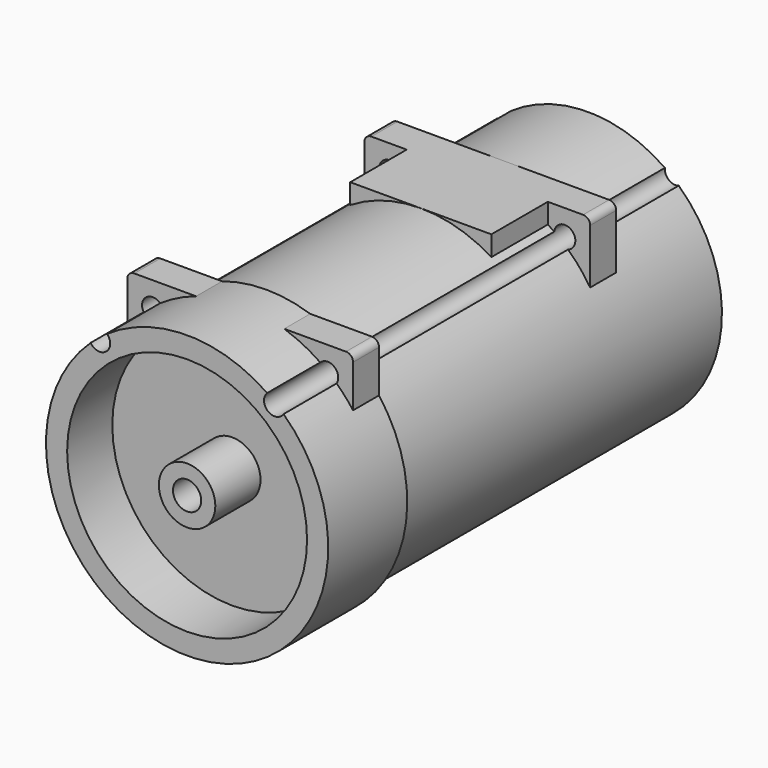
from build123d import *

# Parameters (mm, degrees)
F0_R      = 95
F1_DEPTH  = 355
F3_DEPTH  = 70
F4_R      = 85
F4_R_2    = 20
F5_DEPTH  = 40
F6_R      = 10
F7_DEPTH  = 25
F10_DEPTH = 98
F11_R     = 100
F11_R_2   = 95
F12_DEPTH = 70
F8_R      = 7.5
F13_DEPTH = 500
F14_R     = 5
F16_DEPTH = 47
F18_DEPTH = 75
F19_W     = 100
F19_H     = 50
F20_DEPTH = 22


# Not quite as in the source:
# - a feature names something its author has since deleted; it is built from what else it names


with BuildPart() as f1:
    # F0 (on Front) → F1 (new body)
    with BuildSketch(Plane.XZ):
        Circle(F0_R)
    extrude(amount=F1_DEPTH)

    # F2 (on face) → F3 (join)
    with BuildSketch(Plane.XZ.offset(355)):
        with BuildLine():
            Line((80, 51.2347538298), (80, 95))
            Line((80, 95), (46.4354390525, 95))
            Line((46.4354390525, 95), (0, 95))
            ThreePointArc((0, 95), (45.594398703, 83.3435708793), (80, 51.2347538298))
        make_face()
        with BuildLine():
            ThreePointArc((95, 0), (91.1729126441, 26.6926956301), (80, 51.2347538298))
            Line((80, 51.2347538298), (80, 50))
            Line((80, 50), (-80, 50))
            Line((-80, 50), (-80, 51.2347538298))
            ThreePointArc((-80, 51.2347538298), (-26.6926956301, -91.1729126441), (95, 0))
        make_face()
        with BuildLine():
            Line((80, 50), (80, 51.2347538298))
            ThreePointArc((80, 51.2347538298), (45.594398703, 83.3435708793), (0, 95))
            ThreePointArc((0, 95), (-45.594398703, 83.3435708793), (-80, 51.2347538298))
            Line((-80, 51.2347538298), (-80, 50))
            Line((-80, 50), (80, 50))
        make_face()
        with BuildLine():
            ThreePointArc((-80, 51.2347538298), (-45.594398703, 83.3435708793), (0, 95))
            Line((0, 95), (-46.4354390525, 95))
            Line((-46.4354390525, 95), (-80, 95))
            Line((-80, 95), (-80, 51.2347538298))
        make_face()
    extrude(amount=-F3_DEPTH)

    # F4 (on face) → F5 (cut)
    with BuildSketch(Plane.XZ.offset(355)):
        Circle(F4_R)
        Circle(F4_R_2, mode=Mode.SUBTRACT)
    extrude(amount=-F5_DEPTH, mode=Mode.SUBTRACT)

    # F6 (on face) → F7 (cut)
    with BuildSketch(Plane.XZ.offset(355)):
        Circle(F6_R)
    extrude(amount=-F7_DEPTH, mode=Mode.SUBTRACT)

    # F9 (on face) → F10 (join)
    with BuildSketch(Plane(origin=(0, 0, 0), x_dir=(-1, 0, 0), z_dir=(0, 1, 0))):
        with BuildLine():
            ThreePointArc((-80, 51.2347538298), (-45.594398703, 83.3435708793), (0, 95))
            Line((0, 95), (-75, 95))
            ThreePointArc((-75, 95), (-78.5355339059, 93.5355339059), (-80, 90))
            Line((-80, 90), (-80, 51.2347538298))
        make_face()
        with BuildLine():
            ThreePointArc((0, 95), (45.594398703, 83.3435708793), (80, 51.2347538298))
            Line((80, 51.2347538298), (80, 90))
            ThreePointArc((80, 90), (78.5355339059, 93.5355339059), (75, 95))
            Line((75, 95), (0, 95))
        make_face()
    extrude(amount=-F10_DEPTH)

    # F11 (on face) → F12 (join)
    with BuildSketch(Plane(origin=(0, -285, 0), x_dir=(-1, 0, 0), z_dir=(0, 1, 0))):
        Circle(F11_R)
        Circle(F11_R_2, mode=Mode.SUBTRACT)
    extrude(amount=-F12_DEPTH)

    # F8 (on face) → F13 (cut)
    with BuildSketch(Plane.XZ.offset(355)):
        with Locations((-62, 77)):
            Circle(F8_R)
        with Locations((62, 77)):
            Circle(F8_R)
    extrude(amount=-F13_DEPTH, mode=Mode.SUBTRACT)

    # F14
    f14_edges = [f1.edges().sort_by_distance(p)[0] for p in [
        (-80, -320, 95),
        (80, -320, 95),
    ]]
    fillet(f14_edges, radius=F14_R)

    # F15 (on face) → F16 (cut)
    with BuildSketch(Plane.XZ.offset(355)):
        with BuildLine():
            ThreePointArc((-80, 60), (0, 100), (80, 60))
            Line((80, 60), (80, 108.7283083646))
            Line((80, 108.7283083646), (-80, 108.7283083646))
            Line((-80, 108.7283083646), (-80, 60))
        make_face()
    extrude(amount=-F16_DEPTH, mode=Mode.SUBTRACT)

    # F17 (on face) → F18 (cut)
    with BuildSketch(Plane(origin=(0, 0, 0), x_dir=(-1, 0, 0), z_dir=(0, 1, 0))):
        with BuildLine():
            ThreePointArc((-80, 51.2347538298), (0, 95), (80, 51.2347538298))
            Line((80, 51.2347538298), (80, 103.6055907607))
            Line((80, 103.6055907607), (-80, 103.6055907607))
            Line((-80, 103.6055907607), (-80, 51.2347538298))
        make_face()
    extrude(amount=-F18_DEPTH, mode=Mode.SUBTRACT)

    # F19 (on face) → F20 (join)
    with BuildSketch(Plane.XY.offset(95)):
        with Locations((0, -123)):
            Rectangle(F19_W, F19_H)
    extrude(amount=-F20_DEPTH)


solid = f1.part
